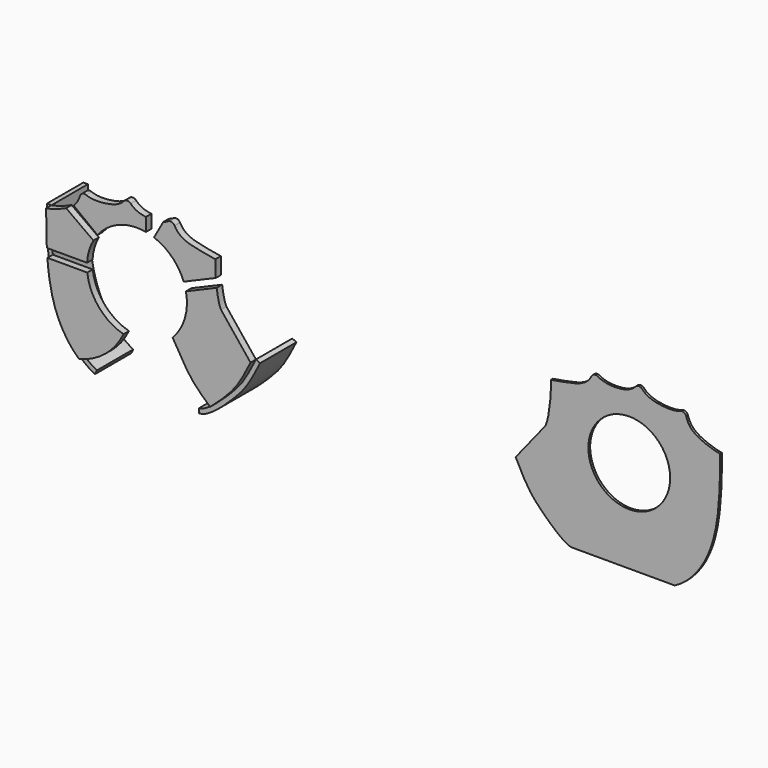
from build123d import *

# Parameters (mm, degrees)
F1_DEPTH = 3.81
F2_DEPTH = 25.4
F0_R     = 22.86
F3_DEPTH = 1.27


# Not quite as in the source:
# - the dataset's text gives a spline's control points without its knots; the knots are read off the source's solid


with BuildPart() as f1:
    # F0 (on Front) → F1 (new body)
    with BuildSketch(Plane.XZ):
        with BuildLine():
            add(Edge.make_bspline(
                [(-32.4015982609, -47.2542967092), (-37.3545101899, -42.8550868765), (-46.2039408348, -30.0827942932), (-49.2886590635, -13.3112173003), (-50.0835223991, -3.1672286712)],
                knots=[0.1324377854, 0.1324377854, 0.1324377854, 0.1324377854, 0.4305745002, 0.7612639779, 0.7612639779, 0.7612639779, 0.7612639779], degree=3))
            ThreePointArc((-32.4015982609, -47.2542967092), (-17.6981427389, -39.8494489219), (-7.5220542761, -26.90840574))
            ThreePointArc((-7.5220542761, -26.90840574), (-21.2629963717, -18.1253575219), (-27.7599038641, -3.1672286712))
            Line((-27.7599038641, -3.1672286712), (-50.0835223991, -3.1672286712))
        make_face()
    extrude(amount=F1_DEPTH)


with BuildPart() as f1b:
    # F0 (on Front) → F1, piece 2 (new body)
    with BuildSketch(Plane.XZ):
        with BuildLine():
            add(Edge.make_bspline(
                [(-50.3942953675, 1.6068994458), (-50.7116523317, 7.6046741304), (-50.8, 14.040708595), (-50.8, 20.955)],
                knots=[0.8121129163, 0.8121129163, 0.8121129163, 0.8121129163, 1, 1, 1, 1], degree=3))
            Line((-50.3942953675, 1.6068994458), (-27.8937533181, 1.6068994458))
            ThreePointArc((-27.8937533181, 1.6068994458), (-26.8082807521, 7.8714473331), (-24.3346381376, 13.728400734))
            Line((-24.3346381376, 13.728400734), (-39.5643113353, 24.685851328))
            add(Edge.make_bspline(
                [(-50.8, 20.955), (-48.7586294455, 21.2383932933), (-43.6710240911, 22.6255829589), (-39.5643113353, 24.685851328)],
                knots=[0, 0, 0, 0, 0.4195234448, 0.4195234448, 0.4195234448, 0.4195234448], degree=3))
        make_face()
    extrude(amount=F1_DEPTH)


with BuildPart() as f1c:
    # F0 (on Front) → F1, piece 3 (new body)
    with BuildSketch(Plane.XZ):
        with BuildLine():
            add(Edge.make_bspline(
                [(19.914929673, -19.5969175158), (23.6612726725, -25.9838738604), (29.5150758275, -36.8834797497), (37.494373544, -43.9061090328), (40.9513666547, -46.9066246366)],
                knots=[0, 0, 0, 0, 0.5400159495, 1, 1, 1, 1], degree=3))
            add(Edge.make_bspline(
                [(40.9513666547, -46.9066246366), (44.1733718974, -44.2593550986), (54.7370471064, -34.0134404836), (57.6018359563, -29.538032362), (63.5, -17.78)],
                knots=[0.2576942768, 0.2576942768, 0.2576942768, 0.2576942768, 0.4906190831, 1, 1, 1, 1], degree=3))
            Line((63.5, -17.78), (46.99, 2.8575))
            add(Edge.make_bspline(
                [(46.99, 2.8575), (45.862430977, 5.0832937801), (45.1728056088, 8.6289787064), (44.6399921579, 12.4485812477), (44.5846144842, 12.8645142485)],
                knots=[0, 0, 0, 0, 0.4365870001, 0.489378166, 0.489378166, 0.489378166, 0.489378166], degree=3))
            Line((44.5846144842, 12.8645142485), (27.3873225339, 5.5297526549))
            ThreePointArc((27.3873225339, 5.5297526549), (26.7808355812, -7.9643232966), (19.914929673, -19.5969175158))
        make_face()
    extrude(amount=F1_DEPTH)


with BuildPart() as f1d:
    # F0 (on Front) → F1, piece 4 (new body)
    with BuildSketch(Plane.XZ):
        with BuildLine():
            add(Edge.make_bspline(
                [(-35.3985657611, 27.4131491477), (-33.5545344545, 29.0862015789), (-32.5238587747, 31.0124628081), (-31.8214549811, 33.2492936319)],
                knots=[0.5850244101, 0.5850244101, 0.5850244101, 0.5850244101, 0.8620266084, 0.8620266084, 0.8620266084, 0.8620266084], degree=3))
            Line((-35.3985657611, 27.4131491477), (-22.0697075917, 17.1339314466))
            ThreePointArc((-22.0697075917, 17.1339314466), (-9.9658017904, 26.1022296878), (5.035185755, 27.4825490887))
            Line((5.035185755, 27.4825490887), (5.035185755, 34.8978384418))
            add(Edge.make_bspline(
                [(-3.5313723507, 38.7236903364), (-1.4189307014, 36.4309038194), (1.5678475341, 35.3090215627), (5.035185755, 34.8978384418)],
                knots=[0.1270665909, 0.1270665909, 0.1270665909, 0.1270665909, 0.4578818969, 0.4578818969, 0.4578818969, 0.4578818969], degree=3))
            ThreePointArc((-3.5313723507, 38.7236903364), (-5.4519924297, 39.5420641845), (-7.337073828, 38.6448544183))
            add(Edge.make_bspline(
                [(-28.4095240871, 34.8280412728), (-25.6780710844, 33.673919279), (-17.1351502938, 33.689358767), (-9.7101082233, 35.8449091476), (-7.337073828, 38.6448544183)],
                knots=[0.1407427733, 0.1407427733, 0.1407427733, 0.1407427733, 0.4904519108, 0.8757713542, 0.8757713542, 0.8757713542, 0.8757713542], degree=3))
            ThreePointArc((-28.4095240871, 34.8280412728), (-30.4647659531, 34.7935107051), (-31.8214549811, 33.2492936319))
        make_face()
    extrude(amount=F1_DEPTH)


with BuildPart() as f1e:
    # F0 (on Front) → F1, piece 5 (new body)
    with BuildSketch(Plane.XZ):
        with BuildLine():
            ThreePointArc((9.5431544801, 26.2596992094), (19.6282702033, 19.8840289888), (26.1339604159, 9.882292901))
            Line((26.1339604159, 9.882292901), (44.0812421649, 17.5375147581))
            add(Edge.make_bspline(
                [(44.0812421649, 17.5375147581), (43.858115131, 20.2905449954), (43.7488704096, 23.2816558809), (43.815, 26.67)],
                knots=[0.6792819517, 0.6792819517, 0.6792819517, 0.6792819517, 1, 1, 1, 1], degree=3))
            add(Edge.make_bspline(
                [(21.0728423917, 35.7919701026), (22.28828545, 33.4127117189), (27.5077311439, 28.806695039), (37.8716832047, 27.8394519795), (43.815, 26.67)],
                knots=[0.1348798284, 0.1348798284, 0.1348798284, 0.1348798284, 0.4426747117, 1, 1, 1, 1], degree=3))
            ThreePointArc((21.0728423917, 35.7919701026), (19.4874893399, 37.084686082), (17.4633046468, 36.7894993108))
            add(Edge.make_bspline(
                [(14.7616470372, 35.5920521842), (15.7595866428, 35.900713839), (16.6759917562, 36.2967184021), (17.4633046468, 36.7894993108)],
                knots=[0.7586250088, 0.7586250088, 0.7586250088, 0.7586250088, 0.8607304966, 0.8607304966, 0.8607304966, 0.8607304966], degree=3))
            Line((14.7616470372, 35.5920521842), (9.5431544801, 26.2596992094))
        make_face()
    extrude(amount=F1_DEPTH)


with BuildPart() as f2:
    # F0 (on Front) → F2 (new body)
    with BuildSketch(Plane.XZ):
        with BuildLine():
            Line((-26.5420038104, -54.3387961377), (-25.4, -52.07))
            add(Edge.make_bspline(
                [(-25.4, -52.07), (-27.8518213277, -50.8358700348), (-30.2014241314, -49.2085062334), (-32.4015982609, -47.2542967092)],
                knots=[0, 0, 0, 0, 0.1324377854, 0.1324377854, 0.1324377854, 0.1324377854], degree=3))
            add(Edge.make_bspline(
                [(-32.4015982609, -47.2542967092), (-37.3545101899, -42.8550868765), (-46.2039408348, -30.0827942932), (-49.2886590635, -13.3112173003), (-50.0835223991, -3.1672286712)],
                knots=[0.1324377854, 0.1324377854, 0.1324377854, 0.1324377854, 0.4305745002, 0.7612639779, 0.7612639779, 0.7612639779, 0.7612639779], degree=3))
            add(Edge.make_bspline(
                [(-50.0835223991, -3.1672286712), (-50.2057456917, -1.6074238163), (-50.308407267, -0.0163120564), (-50.3942953675, 1.6068994458)],
                knots=[0.7612639779, 0.7612639779, 0.7612639779, 0.7612639779, 0.8121129163, 0.8121129163, 0.8121129163, 0.8121129163], degree=3))
            add(Edge.make_bspline(
                [(-50.3942953675, 1.6068994458), (-50.7116523317, 7.6046741304), (-50.8, 14.040708595), (-50.8, 20.955)],
                knots=[0.8121129163, 0.8121129163, 0.8121129163, 0.8121129163, 1, 1, 1, 1], degree=3))
            Line((-50.8, 20.955), (-53.3400016963, 20.955))
            add(Edge.make_bspline(
                [(-26.5420038104, -54.3387961377), (-29.0627100455, -53.0699927941), (-33.8490428694, -49.7994585613), (-39.0421158261, -44.2219190116), (-42.6313614699, -39.0406400188), (-45.0149981604, -34.8367031295), (-47.0641498349, -30.3522635024), (-48.7493698024, -25.6395384607), (-50.1060112231, -20.7011376547), (-51.5244817953, -13.8063144268), (-52.6554809616, -4.5873586327), (-53.2616912763, 7.5172788692), (-53.3400016963, 16.3405741938), (-53.3400016963, 20.955)],
                knots=[0, 0, 0, 0, 0.125, 0.25, 0.3125, 0.375, 0.4375, 0.5, 0.5625, 0.625, 0.75, 0.875, 1, 1, 1, 1], degree=3))
        make_face()
    extrude(amount=-F2_DEPTH)


with BuildPart() as f2b:
    # F0 (on Front) → F2, piece 2 (new body)
    with BuildSketch(Plane.XZ):
        with BuildLine():
            add(Edge.make_bspline(
                [(31.75, -52.07), (33.3163124064, -52.0694765021), (35.5326097167, -50.9220271224), (37.9748498683, -49.1938224865)],
                knots=[0, 0, 0, 0, 0.1846780617, 0.1846780617, 0.1846780617, 0.1846780617], degree=3))
            Line((31.75, -52.07), (31.7508489268, -54.6099998581))
            add(Edge.make_bspline(
                [(31.7508489268, -54.6099998581), (32.2256640176, -54.6098411639), (33.1335262146, -54.4951302851), (34.4187918601, -54.110885336), (35.682925068, -53.5675580748), (37.3779369898, -52.6643683647), (39.5484147263, -51.2417084284), (42.2305963042, -49.1791129251), (44.9257896, -46.8787646379), (47.5528122711, -44.4636194039), (49.6099867185, -42.4609157239), (51.1312464786, -40.9269854625), (52.195470601, -39.8299669872), (53.1852172114, -38.7853468766), (54.4235542152, -37.4350675119), (55.8419358132, -35.7893265179), (57.4065121682, -33.7640279942), (59.3953643105, -30.856502217), (61.8771429381, -26.5786619273), (64.3175942448, -21.8149867836), (65.7703642316, -18.918879386)],
                knots=[0, 0, 0, 0, 0.03125, 0.0625, 0.09375, 0.125, 0.1875, 0.25, 0.3125, 0.375, 0.4375, 0.46875, 0.5, 0.53125, 0.5625, 0.625, 0.6875, 0.75, 0.875, 1, 1, 1, 1], degree=3))
            Line((65.7703642316, -18.918879386), (63.5, -17.78))
            add(Edge.make_bspline(
                [(40.9513666547, -46.9066246366), (44.1733718974, -44.2593550986), (54.7370471064, -34.0134404836), (57.6018359563, -29.538032362), (63.5, -17.78)],
                knots=[0.2576942768, 0.2576942768, 0.2576942768, 0.2576942768, 0.4906190831, 1, 1, 1, 1], degree=3))
            add(Edge.make_bspline(
                [(37.9748498683, -49.1938224865), (38.9404390166, -48.5105417529), (39.9413470189, -47.7364787222), (40.9513666547, -46.9066246366)],
                knots=[0.1846780617, 0.1846780617, 0.1846780617, 0.1846780617, 0.2576942768, 0.2576942768, 0.2576942768, 0.2576942768], degree=3))
        make_face()
    extrude(amount=-F2_DEPTH)


with BuildPart() as f3:
    # F0 (on Front) → F3 (new body)
    with BuildSketch(Plane.XZ):
        with BuildLine():
            ThreePointArc((255.7475026767, 36.7894993108), (253.7233179835, 37.084686082), (252.1379649318, 35.7919701026))
            add(Edge.make_bspline(
                [(252.1379649318, 35.7919701026), (250.9225218734, 33.4127117189), (245.7030761795, 28.806695039), (235.3391241187, 27.8394519795), (229.3958073235, 26.67)],
                knots=[0.1348798284, 0.1348798284, 0.1348798284, 0.1348798284, 0.4426747117, 1, 1, 1, 1], degree=3))
            add(Edge.make_bspline(
                [(226.2208073235, 2.8575), (227.3483763465, 5.0832937801), (228.7575633843, 12.3285800892), (229.5119787429, 20.7176155465), (229.3958073235, 26.67)],
                knots=[0, 0, 0, 0, 0.4365870001, 1, 1, 1, 1], degree=3))
            Line((226.2208073235, 2.8575), (209.7108073235, -17.78))
            add(Edge.make_bspline(
                [(241.4608073235, -52.07), (237.29971342, -52.0686092659), (219.4682826462, -35.5670955658), (215.6089713672, -29.538032362), (209.7108073235, -17.78)],
                knots=[0, 0, 0, 0, 0.4906190831, 1, 1, 1, 1], degree=3))
            Line((241.4608073235, -52.07), (298.6108073235, -52.07))
            add(Edge.make_bspline(
                [(298.6108073235, -52.07), (306.5820350195, -48.0576640078), (322.5857309093, -29.0858098177), (324.0108073235, 0), (324.0108073235, 20.955)],
                knots=[0, 0, 0, 0, 0.4305745002, 1, 1, 1, 1], degree=3))
            add(Edge.make_bspline(
                [(324.0108073235, 20.955), (321.4156890461, 21.315267328), (309.2638781363, 24.7808695382), (305.8657632634, 30.5949790437), (305.0322623045, 33.2492936319)],
                knots=[0, 0, 0, 0, 0.5333245143, 0.8620266084, 0.8620266084, 0.8620266084, 0.8620266084], degree=3))
            ThreePointArc((305.0322623045, 33.2492936319), (303.6755732765, 34.7935107051), (301.6203314105, 34.8280412728))
            add(Edge.make_bspline(
                [(301.6203314105, 34.8280412728), (298.8888784079, 33.673919279), (290.3459576173, 33.689358767), (282.9209155468, 35.8449091476), (280.5478811515, 38.6448544183)],
                knots=[0.1407427733, 0.1407427733, 0.1407427733, 0.1407427733, 0.4904519108, 0.8757713542, 0.8757713542, 0.8757713542, 0.8757713542], degree=3))
            ThreePointArc((280.5478811515, 38.6448544183), (278.6627997531, 39.5420641845), (276.7421796741, 38.7236903364))
            add(Edge.make_bspline(
                [(276.7421796741, 38.7236903364), (274.3984555692, 36.1798761539), (267.5622447281, 33.976136877), (258.5744980657, 35.0200765395), (255.7475026767, 36.7894993108)],
                knots=[0.1270665909, 0.1270665909, 0.1270665909, 0.1270665909, 0.4941014897, 0.8607304966, 0.8607304966, 0.8607304966, 0.8607304966], degree=3))
        make_face()
        with Locations((273.2108073235, 0)):
            Circle(F0_R, mode=Mode.SUBTRACT)
    extrude(amount=F3_DEPTH)


solid = Compound([f1.part, f1b.part, f1c.part, f1d.part, f1e.part, f2.part, f2b.part, f3.part])
